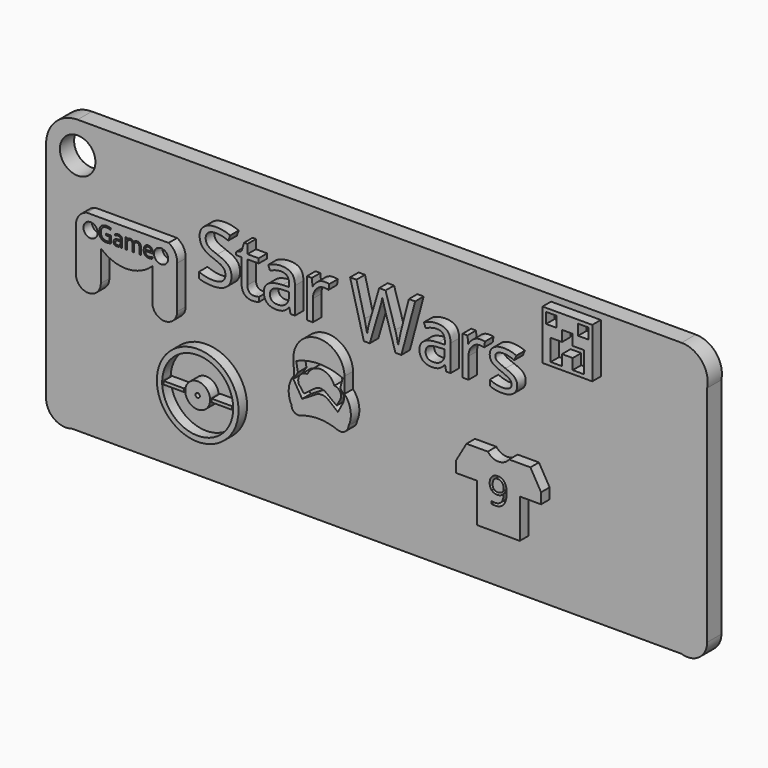
from build123d import *

# Parameters (mm, degrees)
F0_R         = 2.5
F1_DEPTH     = 2.5
F2_R         = 1
F2_W         = 7
F2_H         = 7
F2_W_2       = 1.5
F2_H_2       = 1.5
F3_DEPTH     = 1.5
F4_R         = 5.75
F4_R_2       = 0.3075408847
F4_W         = 2.85
F4_H         = 0.4542748781
F5_DEPTH     = 1.5
F6_TEXT_SIZE = 10.1908371098
F7_DEPTH     = 1.5


# Not quite as in the source:
# - a feature names something its author has since deleted; it is built from what else it names
# - Text() gives the source's letters only with a copy of the font that has no kerning and outlines rounded to 1/6400 em; it was checked with that copy


with BuildPart() as f1:
    # F0 (on Front) → F1 (new body)
    with BuildSketch(Plane.XZ):
        with BuildLine():
            Line((40.1452163594, 33.2882386101), (-44.8547836406, 33.2882386101))
            ThreePointArc((-44.8547836406, 33.2882386101), (-47.9977809885, 31.986366482), (-49.2996531166, 28.8433691341))
            Line((-49.2996531166, 28.8433691341), (-49.2996531166, -2.6566308659))
            ThreePointArc((-49.2996531166, -2.6566308659), (-48.1632971226, -4.8790656039), (-45.6962897411, -5.2590599318))
            Line((-45.6962897411, -5.2590599318), (40.1452163594, -5.2590599318))
            ThreePointArc((40.1452163594, -5.2590599318), (42.6122237409, -4.8790656039), (43.7485797349, -2.6566308659))
            Line((43.7485797349, -2.6566308659), (43.7485797349, 28.8433691341))
            ThreePointArc((43.7485797349, 28.8433691341), (43.0062079827, 31.9245644376), (40.1452163594, 33.2882386101))
        make_face()
        with Locations((-44.8547836406, 28.8433691341)):
            Circle(F0_R, mode=Mode.SUBTRACT)
    extrude(amount=F1_DEPTH)

    # F2 (on face) → F3 (join)
    with BuildSketch(Plane.XZ.offset(2.5)):
        with BuildLine():
            Line((-30.8494087805, 23.1841380224), (-42.3494087805, 23.1841380224))
            ThreePointArc((-42.3494087805, 23.1841380224), (-43.5077424075, 22.3980029631), (-43.8982113336, 21.0536521382))
            Line((-43.8982113336, 21.0536521382), (-43.8982113336, 15.0536521382))
            ThreePointArc((-43.8982113336, 15.0536521382), (-42.1482113336, 13.3036521382), (-40.3982113336, 15.0536521382))
            Line((-40.3982113336, 15.0536521382), (-40.3982113336, 19.422019965))
            ThreePointArc((-40.3982113336, 19.422019965), (-36.749148121, 18.0498369187), (-33.1518526471, 19.5525058492))
            Line((-33.1518526471, 19.5525058492), (-33.1518526471, 15.0536521382))
            ThreePointArc((-33.1518526471, 15.0536521382), (-31.4018526471, 13.3036521382), (-29.6518526471, 15.0536521382))
            Line((-29.6518526471, 15.0536521382), (-29.6518526471, 21.0536521382))
            ThreePointArc((-29.6518526471, 21.0536521382), (-29.9387035959, 22.29423078), (-30.8494087805, 23.1841380224))
        make_face()
        with Locations((-41.8379865587, 21.1841380224)):
            Circle(F2_R, mode=Mode.SUBTRACT)
        with BuildLine():
            Line((-37.3889529858, 20.4051174223), (-37.5595331635, 20.4051174223))
            Line((-37.5595331635, 20.4051174223), (-37.6051688994, 20.6213333359))
            Line((-37.6051688994, 20.6213333359), (-37.6162455343, 20.6213333359))
            add(Edge.make_bspline(
                [(-37.6162455343, 20.6213333359), (-37.7296702758, 20.4786662782), (-37.8424304193, 20.4279352903)],
                knots=[0, 0, 0, 1, 1, 1], degree=2))
            add(Edge.make_bspline(
                [(-37.8424304193, 20.4279352903), (-37.9551905628, 20.3772043023), (-38.1244415443, 20.3772043023)],
                knots=[0, 0, 0, 1, 1, 1], degree=2))
            add(Edge.make_bspline(
                [(-38.1244415443, 20.3772043023), (-38.3499618312, 20.3772043023), (-38.4780077309, 20.4937305017)],
                knots=[0, 0, 0, 1, 1, 1], degree=2))
            add(Edge.make_bspline(
                [(-38.4780077309, 20.4937305017), (-38.6060536305, 20.610256701), (-38.6060536305, 20.824700353)],
                knots=[0, 0, 0, 1, 1, 1], degree=2))
            add(Edge.make_bspline(
                [(-38.6060536305, 20.824700353), (-38.6060536305, 21.2841591694), (-37.8710081374, 21.3063124393)],
                knots=[0, 0, 0, 1, 1, 1], degree=2))
            Line((-37.8710081374, 21.3063124393), (-37.6135871419, 21.3147306818))
            Line((-37.6135871419, 21.3147306818), (-37.6135871419, 21.4091036113))
            add(Edge.make_bspline(
                [(-37.6135871419, 21.4091036113), (-37.6135871419, 21.5876589662), (-37.6902374555, 21.6727275223)],
                knots=[0, 0, 0, 1, 1, 1], degree=2))
            add(Edge.make_bspline(
                [(-37.6902374555, 21.6727275223), (-37.7668877692, 21.7577960785), (-37.9361387507, 21.7577960785)],
                knots=[0, 0, 0, 1, 1, 1], degree=2))
            add(Edge.make_bspline(
                [(-37.9361387507, 21.7577960785), (-38.1257707405, 21.7577960785), (-38.3650260547, 21.6417129446)],
                knots=[0, 0, 0, 1, 1, 1], degree=2))
            Line((-38.3650260547, 21.6417129446), (-38.4359165182, 21.8176099071))
            add(Edge.make_bspline(
                [(-38.4359165182, 21.8176099071), (-38.3238209728, 21.8783098664), (-38.1902367557, 21.9128689674)],
                knots=[0, 0, 0, 1, 1, 1], degree=2))
            add(Edge.make_bspline(
                [(-38.1902367557, 21.9128689674), (-38.0566525386, 21.9474280683), (-37.921960658, 21.9474280683)],
                knots=[0, 0, 0, 1, 1, 1], degree=2))
            add(Edge.make_bspline(
                [(-37.921960658, 21.9474280683), (-37.6508046352, 21.9474280683), (-37.5198788105, 21.8271358131)],
                knots=[0, 0, 0, 1, 1, 1], degree=2))
            add(Edge.make_bspline(
                [(-37.5198788105, 21.8271358131), (-37.3889529858, 21.7068435579), (-37.3889529858, 21.4410043199)],
                knots=[0, 0, 0, 1, 1, 1], degree=2))
            Line((-37.3889529858, 21.4410043199), (-37.3889529858, 20.4051174223))
        make_face(mode=Mode.SUBTRACT)
        with BuildLine():
            Line((-39.6317500239, 21.2553599186), (-39.6317500239, 21.4658159821))
            Line((-39.6317500239, 21.4658159821), (-38.9436694628, 21.4658159821))
            Line((-38.9436694628, 21.4658159821), (-38.9436694628, 20.4813246706))
            add(Edge.make_bspline(
                [(-38.9436694628, 20.4813246706), (-39.1045022019, 20.4299290846), (-39.2706517256, 20.4035666935)],
                knots=[0, 0, 0, 1, 1, 1], degree=2))
            add(Edge.make_bspline(
                [(-39.2706517256, 20.4035666935), (-39.4368012494, 20.3772043023), (-39.6556755554, 20.3772043023)],
                knots=[0, 0, 0, 1, 1, 1], degree=2))
            add(Edge.make_bspline(
                [(-39.6556755554, 20.3772043023), (-40.1151343718, 20.3772043023), (-40.3712261711, 20.6507971848)],
                knots=[0, 0, 0, 1, 1, 1], degree=2))
            add(Edge.make_bspline(
                [(-40.3712261711, 20.6507971848), (-40.6273179704, 20.9243900673), (-40.6273179704, 21.4170787884)],
                knots=[0, 0, 0, 1, 1, 1], degree=2))
            add(Edge.make_bspline(
                [(-40.6273179704, 21.4170787884), (-40.6273179704, 21.7329844163), (-40.5006012669, 21.9704674689)],
                knots=[0, 0, 0, 1, 1, 1], degree=2))
            add(Edge.make_bspline(
                [(-40.5006012669, 21.9704674689), (-40.3738845635, 22.2079505216), (-40.1357369127, 22.3331164962)],
                knots=[0, 0, 0, 1, 1, 1], degree=2))
            add(Edge.make_bspline(
                [(-40.1357369127, 22.3331164962), (-39.897589262, 22.4582824707), (-39.5781391109, 22.4582824707)],
                knots=[0, 0, 0, 1, 1, 1], degree=2))
            add(Edge.make_bspline(
                [(-39.5781391109, 22.4582824707), (-39.2538152406, 22.4582824707), (-38.9742409752, 22.3395409444)],
                knots=[0, 0, 0, 1, 1, 1], degree=2))
            Line((-38.9742409752, 22.3395409444), (-39.0655124469, 22.1317432733))
            add(Edge.make_bspline(
                [(-39.0655124469, 22.1317432733), (-39.3397699275, 22.2478264073), (-39.5932033344, 22.2478264073)],
                knots=[0, 0, 0, 1, 1, 1], degree=2))
            add(Edge.make_bspline(
                [(-39.5932033344, 22.2478264073), (-39.9627198753, 22.2478264073), (-40.1705175464, 22.0278444378)],
                knots=[0, 0, 0, 1, 1, 1], degree=2))
            add(Edge.make_bspline(
                [(-40.1705175464, 22.0278444378), (-40.3783152174, 21.8078624683), (-40.3783152174, 21.4170787884)],
                knots=[0, 0, 0, 1, 1, 1], degree=2))
            add(Edge.make_bspline(
                [(-40.3783152174, 21.4170787884), (-40.3783152174, 21.0072432965), (-40.1782711908, 20.7954580369)],
                knots=[0, 0, 0, 1, 1, 1], degree=2))
            add(Edge.make_bspline(
                [(-40.1782711908, 20.7954580369), (-39.9782271642, 20.5836727772), (-39.5905449421, 20.5836727772)],
                knots=[0, 0, 0, 1, 1, 1], degree=2))
            add(Edge.make_bspline(
                [(-39.5905449421, 20.5836727772), (-39.3800888786, 20.5836727772), (-39.1793802539, 20.6324099709)],
                knots=[0, 0, 0, 1, 1, 1], degree=2))
            Line((-39.1793802539, 20.6324099709), (-39.1793802539, 21.2553599186))
            Line((-39.1793802539, 21.2553599186), (-39.6317500239, 21.2553599186))
        make_face(mode=Mode.SUBTRACT)
        with BuildLine():
            Line((-34.7518277445, 20.4051174223), (-34.98133562, 20.4051174223))
            Line((-34.98133562, 20.4051174223), (-34.98133562, 21.3922671262))
            add(Edge.make_bspline(
                [(-34.98133562, 21.3922671262), (-34.98133562, 21.5739239389), (-35.0588720644, 21.6645308125)],
                knots=[0, 0, 0, 1, 1, 1], degree=2))
            add(Edge.make_bspline(
                [(-35.0588720644, 21.6645308125), (-35.1364085089, 21.7551376861), (-35.2998996402, 21.7551376861)],
                knots=[0, 0, 0, 1, 1, 1], degree=2))
            add(Edge.make_bspline(
                [(-35.2998996402, 21.7551376861), (-35.5143432923, 21.7551376861), (-35.6169129316, 21.6319655059)],
                knots=[0, 0, 0, 1, 1, 1], degree=2))
            add(Edge.make_bspline(
                [(-35.6169129316, 21.6319655059), (-35.7194825709, 21.5087933256), (-35.7194825709, 21.2527015263)],
                knots=[0, 0, 0, 1, 1, 1], degree=2))
            Line((-35.7194825709, 21.2527015263), (-35.7194825709, 20.4051174223))
            Line((-35.7194825709, 20.4051174223), (-35.9494335118, 20.4051174223))
            Line((-35.9494335118, 20.4051174223), (-35.9494335118, 21.3922671262))
            add(Edge.make_bspline(
                [(-35.9494335118, 21.3922671262), (-35.9494335118, 21.5739239389), (-36.0269699563, 21.6645308125)],
                knots=[0, 0, 0, 1, 1, 1], degree=2))
            add(Edge.make_bspline(
                [(-36.0269699563, 21.6645308125), (-36.1045064007, 21.7551376861), (-36.2693267283, 21.7551376861)],
                knots=[0, 0, 0, 1, 1, 1], degree=2))
            add(Edge.make_bspline(
                [(-36.2693267283, 21.7551376861), (-36.4850995765, 21.7551376861), (-36.5854538888, 21.6257625903)],
                knots=[0, 0, 0, 1, 1, 1], degree=2))
            add(Edge.make_bspline(
                [(-36.5854538888, 21.6257625903), (-36.6858082012, 21.4963874945), (-36.6858082012, 21.2013059402)],
                knots=[0, 0, 0, 1, 1, 1], degree=2))
            Line((-36.6858082012, 21.2013059402), (-36.6858082012, 20.4051174223))
            Line((-36.6858082012, 20.4051174223), (-36.9157591421, 20.4051174223))
            Line((-36.9157591421, 20.4051174223), (-36.9157591421, 21.9226164061))
            Line((-36.9157591421, 21.9226164061), (-36.7287855447, 21.9226164061))
            Line((-36.7287855447, 21.9226164061), (-36.6915680513, 21.714818735))
            Line((-36.6915680513, 21.714818735), (-36.6804914164, 21.714818735))
            add(Edge.make_bspline(
                [(-36.6804914164, 21.714818735), (-36.6153608031, 21.8255850842), (-36.4968408095, 21.8880573052)],
                knots=[0, 0, 0, 1, 1, 1], degree=2))
            add(Edge.make_bspline(
                [(-36.4968408095, 21.8880573052), (-36.3783208159, 21.9505295261), (-36.2316661695, 21.9505295261)],
                knots=[0, 0, 0, 1, 1, 1], degree=2))
            add(Edge.make_bspline(
                [(-36.2316661695, 21.9505295261), (-35.875884656, 21.9505295261), (-35.766447503, 21.6926654652)],
                knots=[0, 0, 0, 1, 1, 1], degree=2))
            Line((-35.766447503, 21.6926654652), (-35.7553708681, 21.6926654652))
            add(Edge.make_bspline(
                [(-35.7553708681, 21.6926654652), (-35.6875818624, 21.8118500569), (-35.5588713646, 21.8811897915)],
                knots=[0, 0, 0, 1, 1, 1], degree=2))
            add(Edge.make_bspline(
                [(-35.5588713646, 21.8811897915), (-35.4301608669, 21.9505295261), (-35.2653405393, 21.9505295261)],
                knots=[0, 0, 0, 1, 1, 1], degree=2))
            add(Edge.make_bspline(
                [(-35.2653405393, 21.9505295261), (-35.0079195438, 21.9505295261), (-34.8798736442, 21.8182745052)],
                knots=[0, 0, 0, 1, 1, 1], degree=2))
            add(Edge.make_bspline(
                [(-34.8798736442, 21.8182745052), (-34.7518277445, 21.6860194843), (-34.7518277445, 21.3949255186)],
                knots=[0, 0, 0, 1, 1, 1], degree=2))
            Line((-34.7518277445, 21.3949255186), (-34.7518277445, 20.4051174223))
        make_face(mode=Mode.SUBTRACT)
        with BuildLine():
            add(Edge.make_bspline(
                [(-33.3747804915, 20.400243703), (-33.4833315137, 20.3772043023), (-33.6370752064, 20.3772043023)],
                knots=[0, 0, 0, 1, 1, 1], degree=2))
            add(Edge.make_bspline(
                [(-33.6370752064, 20.3772043023), (-33.9733618425, 20.3772043023), (-34.1680890843, 20.582343581)],
                knots=[0, 0, 0, 1, 1, 1], degree=2))
            add(Edge.make_bspline(
                [(-34.1680890843, 20.582343581), (-34.3628163262, 20.7874828597), (-34.3628163262, 21.1512395504)],
                knots=[0, 0, 0, 1, 1, 1], degree=2))
            add(Edge.make_bspline(
                [(-34.3628163262, 21.1512395504), (-34.3628163262, 21.5185407643), (-34.1820456443, 21.7345351452)],
                knots=[0, 0, 0, 1, 1, 1], degree=2))
            add(Edge.make_bspline(
                [(-34.1820456443, 21.7345351452), (-34.0012749625, 21.9505295261), (-33.6964459695, 21.9505295261)],
                knots=[0, 0, 0, 1, 1, 1], degree=2))
            add(Edge.make_bspline(
                [(-33.6964459695, 21.9505295261), (-33.4115549194, 21.9505295261), (-33.2454053957, 21.7628913306)],
                knots=[0, 0, 0, 1, 1, 1], degree=2))
            add(Edge.make_bspline(
                [(-33.2454053957, 21.7628913306), (-33.0792558719, 21.5752531351), (-33.0792558719, 21.2677657498)],
                knots=[0, 0, 0, 1, 1, 1], degree=2))
            Line((-33.0792558719, 21.2677657498), (-33.0792558719, 21.1224402996))
            Line((-33.0792558719, 21.1224402996), (-34.1244471428, 21.1224402996))
            add(Edge.make_bspline(
                [(-34.1244471428, 21.1224402996), (-34.1173580964, 20.8552718654), (-33.9893121968, 20.7168139289)],
                knots=[0, 0, 0, 1, 1, 1], degree=2))
            add(Edge.make_bspline(
                [(-33.9893121968, 20.7168139289), (-33.8612662971, 20.5783559925), (-33.6286569638, 20.5783559925)],
                knots=[0, 0, 0, 1, 1, 1], degree=2))
            add(Edge.make_bspline(
                [(-33.6286569638, 20.5783559925), (-33.3836417994, 20.5783559925), (-33.1443864852, 20.6807040991)],
                knots=[0, 0, 0, 1, 1, 1], degree=2))
            Line((-33.1443864852, 20.6807040991), (-33.1443864852, 20.4755648204))
            add(Edge.make_bspline(
                [(-33.1443864852, 20.4755648204), (-33.2662294693, 20.4232831036), (-33.3747804915, 20.400243703)],
                knots=[0, 0, 0, 1, 1, 1], degree=2))
        make_face(mode=Mode.SUBTRACT)
        with Locations((-31.9135896862, 21.1841380224)):
            Circle(F2_R, mode=Mode.SUBTRACT)
        with Locations((25.2758696526, 28.9153070748)):
            Rectangle(F2_W, F2_H)
        Polygon((24.5258696526, 28.9153070748), (24.5258696526, 30.4153070748), (26.0258696526, 30.4153070748), (26.0258696526, 28.9153070748), (27.6258696526, 28.9153070748), (27.6258696526, 25.9153070748), (26.0258696526, 25.9153070748), (26.0258696526, 27.4153070748), (24.5258696526, 27.4153070748), (24.5258696526, 25.9153070748), (22.9258696526, 25.9153070748), (22.9258696526, 28.9153070748), align=None, mode=Mode.SUBTRACT)
        with Locations((23.0258696526, 31.1653070748)):
            Rectangle(F2_W_2, F2_H_2, mode=Mode.SUBTRACT)
        with Locations((27.5258696526, 31.1653070748)):
            Rectangle(F2_W_2, F2_H_2, mode=Mode.SUBTRACT)
        with BuildLine():
            add(Edge.make_bspline(
                [(-38.2897049373, 20.6321884382), (-38.2143838199, 20.5672793575), (-38.0788058085, 20.5672793575)],
                knots=[0, 0, 0, 1, 1, 1], degree=2))
            add(Edge.make_bspline(
                [(-38.0788058085, 20.5672793575), (-37.863919091, 20.5672793575), (-37.7414115089, 20.6849132204)],
                knots=[0, 0, 0, 1, 1, 1], degree=2))
            add(Edge.make_bspline(
                [(-37.7414115089, 20.6849132204), (-37.6189039267, 20.8025470832), (-37.6189039267, 21.0143323428)],
                knots=[0, 0, 0, 1, 1, 1], degree=2))
            Line((-37.6189039267, 21.0143323428), (-37.6189039267, 21.1512395504))
            Line((-37.6189039267, 21.1512395504), (-37.8488548676, 21.1419351771))
            add(Edge.make_bspline(
                [(-37.8488548676, 21.1419351771), (-38.1231123481, 21.1321877384), (-38.2440692014, 21.0566450882)],
                knots=[0, 0, 0, 1, 1, 1], degree=2))
            add(Edge.make_bspline(
                [(-38.2440692014, 21.0566450882), (-38.3650260547, 20.9811024381), (-38.3650260547, 20.8220419607)],
                knots=[0, 0, 0, 1, 1, 1], degree=2))
            add(Edge.make_bspline(
                [(-38.3650260547, 20.8220419607), (-38.3650260547, 20.6970975188), (-38.2897049373, 20.6321884382)],
                knots=[0, 0, 0, 1, 1, 1], degree=2))
        make_face()
        with BuildLine():
            add(Edge.make_bspline(
                [(-33.4224100217, 21.64215601), (-33.5192198108, 21.7577960785), (-33.6995474273, 21.7577960785)],
                knots=[0, 0, 0, 1, 1, 1], degree=2))
            add(Edge.make_bspline(
                [(-33.6995474273, 21.7577960785), (-33.8820903708, 21.7577960785), (-33.9908629256, 21.6388330195)],
                knots=[0, 0, 0, 1, 1, 1], degree=2))
            add(Edge.make_bspline(
                [(-33.9908629256, 21.6388330195), (-34.0996354805, 21.5198699605), (-34.119130358, 21.309413897)],
                knots=[0, 0, 0, 1, 1, 1], degree=2))
            Line((-34.119130358, 21.309413897), (-33.3256002325, 21.309413897))
            add(Edge.make_bspline(
                [(-33.3256002325, 21.309413897), (-33.3256002325, 21.5265159414), (-33.4224100217, 21.64215601)],
                knots=[0, 0, 0, 1, 1, 1], degree=2))
        make_face()
    extrude(amount=F3_DEPTH)

    # F4 (on face) → F5 (join)
    with BuildSketch(Plane.XZ.offset(2.5)):
        with BuildLine():
            Line((14.0738889869, 11.9312809049), (11.0738889869, 11.9312809049))
            Line((11.0738889869, 11.9312809049), (9.5738889869, 9.3332046936))
            Line((9.5738889869, 9.3332046936), (9.5738889869, 7.8332046936))
            Line((9.5738889869, 7.8332046936), (12.5738889869, 7.8332046936))
            Line((12.5738889869, 7.8332046936), (12.5738889869, 2.3332046936))
            Line((12.5738889869, 2.3332046936), (18.5738889869, 2.3332046936))
            Line((18.5738889869, 2.3332046936), (18.5738889869, 7.8332046936))
            Line((18.5738889869, 7.8332046936), (21.5738889869, 7.8332046936))
            Line((21.5738889869, 7.8332046936), (21.5738889869, 9.3332046936))
            Line((21.5738889869, 9.3332046936), (20.0738889869, 11.9312809049))
            Line((20.0738889869, 11.9312809049), (17.0738889869, 11.9312809049))
            ThreePointArc((17.0738889869, 11.9312809049), (15.5738889869, 11.1793509607), (14.0738889869, 11.9312809049))
        make_face()
        with BuildLine():
            add(Edge.make_bspline(
                [(16.589434417, 8.6018994135), (16.7401982873, 8.23403557), (16.7401982873, 7.7339015577)],
                knots=[0, 0, 0, 1, 1, 1], degree=2))
            add(Edge.make_bspline(
                [(16.7401982873, 7.7339015577), (16.7401982873, 5.5773751573), (15.0717447896, 5.5773751573)],
                knots=[0, 0, 0, 1, 1, 1], degree=2))
            add(Edge.make_bspline(
                [(15.0717447896, 5.5773751573), (14.7798659367, 5.5773751573), (14.6094022541, 5.6280318177)],
                knots=[0, 0, 0, 1, 1, 1], degree=2))
            Line((14.6094022541, 5.6280318177), (14.6094022541, 5.9874528844))
            add(Edge.make_bspline(
                [(14.6094022541, 5.9874528844), (14.8104207478, 5.9223228925), (15.0661162718, 5.9223228925)],
                knots=[0, 0, 0, 1, 1, 1], degree=2))
            add(Edge.make_bspline(
                [(15.0661162718, 5.9223228925), (15.6691717529, 5.9223228925), (15.9771320852, 6.2954132168)],
                knots=[0, 0, 0, 1, 1, 1], degree=2))
            add(Edge.make_bspline(
                [(15.9771320852, 6.2954132168), (16.2850924176, 6.6685035411), (16.3124309327, 7.4396104829)],
                knots=[0, 0, 0, 1, 1, 1], degree=2))
            Line((16.3124309327, 7.4396104829), (16.2826801956, 7.4396104829))
            add(Edge.make_bspline(
                [(16.2826801956, 7.4396104829), (16.144379472, 7.2313553234), (15.9156204261, 7.1220012629)],
                knots=[0, 0, 0, 1, 1, 1], degree=2))
            add(Edge.make_bspline(
                [(15.9156204261, 7.1220012629), (15.6868613803, 7.0126472023), (15.4006110453, 7.0126472023)],
                knots=[0, 0, 0, 1, 1, 1], degree=2))
            add(Edge.make_bspline(
                [(15.4006110453, 7.0126472023), (14.9133422165, 7.0126472023), (14.6266898445, 7.3041240182)],
                knots=[0, 0, 0, 1, 1, 1], degree=2))
            add(Edge.make_bspline(
                [(14.6266898445, 7.3041240182), (14.3400374725, 7.595600834), (14.3400374725, 8.1182489176)],
                knots=[0, 0, 0, 1, 1, 1], degree=2))
            add(Edge.make_bspline(
                [(14.3400374725, 8.1182489176), (14.3400374725, 8.6907495877), (14.6604609515, 9.0224301023)],
                knots=[0, 0, 0, 1, 1, 1], degree=2))
            add(Edge.make_bspline(
                [(14.6604609515, 9.0224301023), (14.9808844304, 9.3541106169), (15.5035325141, 9.3541106169)],
                knots=[0, 0, 0, 1, 1, 1], degree=2))
            add(Edge.make_bspline(
                [(15.5035325141, 9.3541106169), (15.8782309863, 9.3541106169), (16.1584507665, 9.1619369369)],
                knots=[0, 0, 0, 1, 1, 1], degree=2))
            add(Edge.make_bspline(
                [(16.1584507665, 9.1619369369), (16.4386705468, 8.969763257), (16.589434417, 8.6018994135)],
                knots=[0, 0, 0, 1, 1, 1], degree=2))
        make_face(mode=Mode.SUBTRACT)
        with BuildLine():
            add(Edge.make_bspline(
                [(15.9268774618, 8.8696560471), (15.7423424846, 8.9979058461), (15.5035325141, 8.9979058461)],
                knots=[0, 0, 0, 1, 1, 1], degree=2))
            add(Edge.make_bspline(
                [(15.5035325141, 8.9979058461), (15.1441114473, 8.9979058461), (14.9483194345, 8.7667345783)],
                knots=[0, 0, 0, 1, 1, 1], degree=2))
            add(Edge.make_bspline(
                [(14.9483194345, 8.7667345783), (14.7525274216, 8.5355633106), (14.7525274216, 8.1230733615)],
                knots=[0, 0, 0, 1, 1, 1], degree=2))
            add(Edge.make_bspline(
                [(14.7525274216, 8.1230733615), (14.7525274216, 7.7612400728), (14.9334440659, 7.5541910243)],
                knots=[0, 0, 0, 1, 1, 1], degree=2))
            add(Edge.make_bspline(
                [(14.9334440659, 7.5541910243), (15.1143607102, 7.3471419758), (15.4834306647, 7.3471419758)],
                knots=[0, 0, 0, 1, 1, 1], degree=2))
            add(Edge.make_bspline(
                [(15.4834306647, 7.3471419758), (15.7125917475, 7.3471419758), (15.9047654275, 7.4400125199)],
                knots=[0, 0, 0, 1, 1, 1], degree=2))
            add(Edge.make_bspline(
                [(15.9047654275, 7.4400125199), (16.0969391075, 7.532883064), (16.207499279, 7.6936978589)],
                knots=[0, 0, 0, 1, 1, 1], degree=2))
            add(Edge.make_bspline(
                [(16.207499279, 7.6936978589), (16.3180594505, 7.8545126539), (16.3180594505, 8.0306048544)],
                knots=[0, 0, 0, 1, 1, 1], degree=2))
            add(Edge.make_bspline(
                [(16.3180594505, 8.0306048544), (16.3180594505, 8.2943411181), (16.2147359448, 8.5178736831)],
                knots=[0, 0, 0, 1, 1, 1], degree=2))
            add(Edge.make_bspline(
                [(16.2147359448, 8.5178736831), (16.111412439, 8.7414062481), (15.9268774618, 8.8696560471)],
                knots=[0, 0, 0, 1, 1, 1], degree=2))
        make_face()
        with Locations((-26.7620570958, 5.6160511449)):
            Circle(F4_R)
        with BuildLine():
            ThreePointArc((-21.7676189727, 5.8518218707), (-21.7634477584, 5.7339693047), (-21.7620570958, 5.6160511449))
            ThreePointArc((-21.7620570958, 5.6160511449), (-26.8799752555, 0.6174418075), (-31.7564952188, 5.8518218707))
            ThreePointArc((-31.7564952188, 5.8518218707), (-26.7620570958, 10.6160511449), (-21.7676189727, 5.8518218707))
        make_face(mode=Mode.SUBTRACT)
        with BuildLine():
            Line((-28.4983623499, 5.8345552972), (-28.4983623499, 5.3975469926))
            ThreePointArc((-28.4983623499, 5.3975469926), (-26.7620570958, 3.8660511449), (-25.0257518417, 5.3975469926))
            Line((-25.0257518417, 5.3975469926), (-25.0257518417, 5.8345552972))
            ThreePointArc((-25.0257518417, 5.8345552972), (-26.7620570958, 7.3660511449), (-28.4983623499, 5.8345552972))
        make_face()
        with Locations((-26.7620570958, 5.6160511449)):
            Circle(F4_R_2, mode=Mode.SUBTRACT)
        with Locations((-30.1370570958, 5.6246844316)):
            Rectangle(F4_W, F4_H)
        with BuildLine():
            ThreePointArc((-28.4983623499, 5.8345552972), (-28.5120570958, 5.6160511449), (-28.4983623499, 5.3975469926))
            Line((-28.4983623499, 5.3975469926), (-28.4983623499, 5.8345552972))
        make_face()
        with Locations((-23.3870570958, 5.6246844316)):
            Rectangle(F4_W, F4_H)
    extrude(amount=F5_DEPTH)

    # F6 (on face) → F7 (join)
    with BuildSketch(Plane.XZ.offset(2.5)):
        with Locations((-27.1095408658, 19.9465118514)):
            Text('Star Wars', F6_TEXT_SIZE, font='Open Sans', text_align=(TextAlign.LEFT, TextAlign.BOTTOM))
        with BuildLine():
            Line((-6.0967034786, 12.5150490803), (-6.0967034786, 14.7093497297))
            ThreePointArc((-6.0967034786, 14.7093497297), (-9.795393421, 18.2113293918), (-13.2973730832, 14.5126394494))
            Line((-13.2973730832, 14.5126394494), (-13.1780909959, 12.5150490803))
            ThreePointArc((-13.1780909959, 12.5150490803), (-13.9369238102, 10.682972967), (-13.5612327132, 8.7358760704))
            ThreePointArc((-13.5612327132, 8.7358760704), (-13.204042884, 7.9812519057), (-12.3925075217, 7.7851586629))
            ThreePointArc((-12.3925075217, 7.7851586629), (-9.6703871492, 8.2648609357), (-6.9633115614, 7.7064745508))
            ThreePointArc((-6.9633115614, 7.7064745508), (-6.0115726545, 7.8918427776), (-5.5279980957, 8.7322736031))
            ThreePointArc((-5.5279980957, 8.7322736031), (-5.2411638942, 10.7095340198), (-6.0967034786, 12.5150490803))
        make_face()
        with BuildLine():
            Line((-13.2973730832, 12.029562045), (-12.6471593814, 13.0598450402))
            Line((-12.6471593814, 13.0598450402), (-12.8973730832, 14.4050199621))
            ThreePointArc((-12.8973730832, 14.4050199621), (-9.6268298374, 15.0885940447), (-6.3562865917, 14.4050199621))
            Line((-6.3562865917, 14.4050199621), (-6.6862354122, 13.0598450402))
            Line((-6.6862354122, 13.0598450402), (-6.1431894468, 12.1968506485))
            Line((-6.1431894468, 12.1968506485), (-6.2158137922, 11.5144201155))
            Line((-6.2158137922, 11.5144201155), (-7.0173977109, 9.9689951908))
            Line((-7.0173977109, 9.9689951908), (-8.3420473379, 11.0356013943))
            ThreePointArc((-8.3420473379, 11.0356013943), (-9.313268419, 11.3780127144), (-10.2844895001, 11.0356013943))
            Line((-10.2844895001, 11.0356013943), (-12.0584261178, 9.9689951908))
            Line((-12.0584261178, 9.9689951908), (-13.2973730832, 12.029562045))
        make_face(mode=Mode.SUBTRACT)
        with BuildLine():
            ThreePointArc((-6.6862354122, 11.6616036474), (-6.7164870213, 12.598532356), (-7.5325392085, 13.0598450402))
            ThreePointArc((-7.5325392085, 13.0598450402), (-9.3505094908, 14.4923199914), (-11.3225093225, 13.2806199061))
            ThreePointArc((-11.3225093225, 13.2806199061), (-12.3711306621, 12.8022293703), (-12.5367723803, 11.6616036474))
            Line((-12.5367723803, 11.6616036474), (-11.8008547212, 10.7049119862))
            Line((-11.8008547212, 10.7049119862), (-10.2554306603, 11.8455828462))
            ThreePointArc((-10.2554306603, 11.8455828462), (-9.4827181979, 12.1048251647), (-8.7100057356, 11.8455828462))
            Line((-8.7100057356, 11.8455828462), (-7.2013769098, 10.7049119862))
            Line((-7.2013769098, 10.7049119862), (-6.6862354122, 11.6616036474))
        make_face()
    extrude(amount=F7_DEPTH)


solid = f1.part
